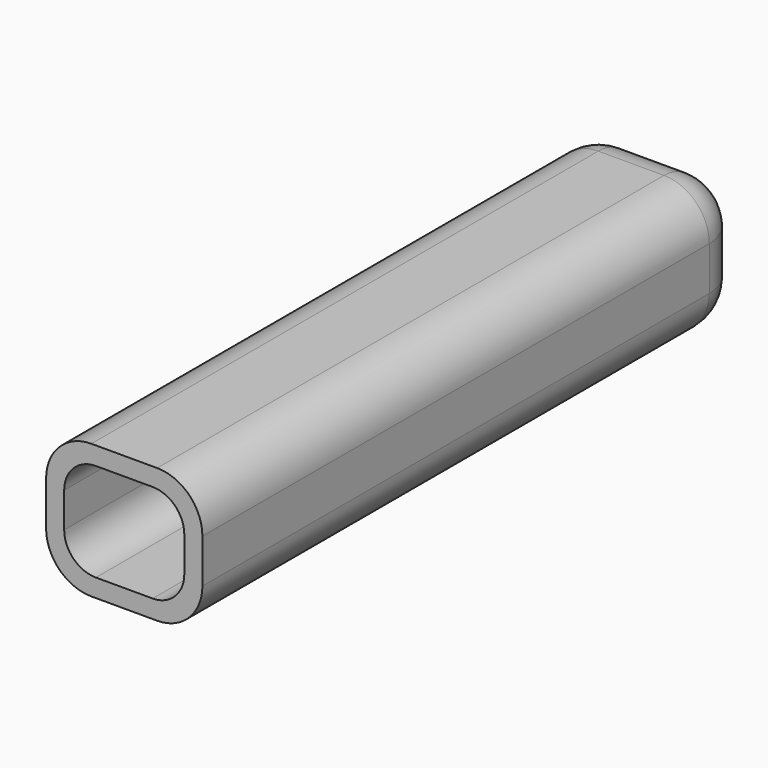
from build123d import *

# Parameters (mm, degrees)
F0_W         = 17.27
F0_H         = 14.85
F0_W_2       = 13.27
F0_H_2       = 10.85
F1_DEPTH     = 75
F2_R         = 3.5
F3_R         = 5
F4_W         = 13.27
F4_H         = 10.85
F5_DEPTH     = 5
F6_R         = 3
F7_DEPTH     = 25
F8_T1_DEPTH  = 7.27
F8_T3_DEPTH  = 4.85
F8_T6_ANGLE  = 90
F8_T8_ANGLE  = 90
F8_T10_ANGLE = 90
F8_T12_ANGLE = 90


# Not quite as in the source:
# - a fillet or chamfer that OpenCascade refuses, or shapes differently, is made with other operations: its cross-section is extruded or revolved along the edge and cut away or added


with BuildPart() as f1:
    # F0 (on Front) → F1 (new body)
    with BuildSketch(Plane.XZ):
        with Locations((6.635, 5.425)):
            Rectangle(F0_W, F0_H)
        with Locations((6.635, 5.425)):
            Rectangle(F0_W_2, F0_H_2, mode=Mode.SUBTRACT)
    extrude(amount=F1_DEPTH)

    # F2
    f2_edges = [f1.edges().sort_by_distance(p)[0] for p in [
        (0, -37.5, 10.85),
        (13.27, -37.5, 0),
        (13.27, -37.5, 10.85),
        (0, -37.5, 0),
    ]]
    fillet(f2_edges, radius=F2_R)

    # F3
    f3_edges = [f1.edges().sort_by_distance(p)[0] for p in [
        (-2, -37.5, 12.85),
        (15.27, -37.5, 12.85),
        (15.27, -37.5, -2),
        (-2, -37.5, -2),
    ]]
    fillet(f3_edges, radius=F3_R)

    # F4 (on face) → F5 (join)
    with BuildSketch(Plane.XZ):
        with Locations((6.635, 5.425)):
            Rectangle(F4_W, F4_H)
    extrude(amount=F5_DEPTH)

    # F6 (on face) → F7 (cut)
    with BuildSketch(Plane.XZ):
        with Locations((6.635, 5.425)):
            Circle(F6_R)
    extrude(amount=F7_DEPTH, mode=Mode.SUBTRACT)

    # F8: fillet of radius 5 on 8 edges, made by hand

    # F8_s2 → F8_t1 (cut)
    with BuildSketch(Plane.YZ.offset(3)):
        with BuildLine():
            ThreePointArc((0, 7.85), (-1.4644660941, 11.3855339059), (-5, 12.85))
            Line((-5, 12.85), (0, 12.85))
            Line((0, 12.85), (0, 7.85))
        make_face()
        with BuildLine():
            ThreePointArc((0, 3), (-1.4644660941, -0.5355339059), (-5, -2))
            Line((-5, -2), (0, -2))
            Line((0, -2), (0, 3))
        make_face()
    extrude(amount=F8_T1_DEPTH, mode=Mode.SUBTRACT)

    # F8_s4 → F8_t3 (cut)
    with BuildSketch(Plane.XY.offset(3)):
        with BuildLine():
            ThreePointArc((3, 0), (-0.5355339059, -1.4644660941), (-2, -5))
            Line((-2, -5), (-2, 0))
            Line((-2, 0), (3, 0))
        make_face()
        with BuildLine():
            ThreePointArc((10.27, 0), (13.8055339059, -1.4644660941), (15.27, -5))
            Line((15.27, -5), (15.27, 0))
            Line((15.27, 0), (10.27, 0))
        make_face()
    extrude(amount=F8_T3_DEPTH, mode=Mode.SUBTRACT)

    # F8_s5 → F8_t6 (revolve, cut)
    with BuildSketch(Plane.XY.offset(7.85)):
        with BuildLine():
            ThreePointArc((3, 0), (-0.5355339059, -1.4644660941), (-2, -5))
            Line((-2, -5), (-2, 0))
            Line((-2, 0), (3, 0))
        make_face()
    revolve(axis=Axis((3, 0, 7.85), (0, 1, 0)), revolution_arc=F8_T6_ANGLE, mode=Mode.SUBTRACT)

    # F8_s7 → F8_t8 (revolve, cut)
    with BuildSketch(Plane.XY.offset(3)):
        with BuildLine():
            ThreePointArc((3, 0), (-0.5355339059, -1.4644660941), (-2, -5))
            Line((-2, -5), (-2, 0))
            Line((-2, 0), (3, 0))
        make_face()
    revolve(axis=Axis((3, 0, 3), (0, -1, 0)), revolution_arc=F8_T8_ANGLE, mode=Mode.SUBTRACT)

    # F8_s9 → F8_t10 (revolve, cut)
    with BuildSketch(Plane.XY.offset(7.85)):
        with BuildLine():
            ThreePointArc((10.27, 0), (13.8055339059, -1.4644660941), (15.27, -5))
            Line((15.27, -5), (15.27, 0))
            Line((15.27, 0), (10.27, 0))
        make_face()
    revolve(axis=Axis((10.27, 0, 7.85), (0, -1, 0)), revolution_arc=F8_T10_ANGLE, mode=Mode.SUBTRACT)

    # F8_s11 → F8_t12 (revolve, cut)
    with BuildSketch(Plane.YZ.offset(10.27)):
        with BuildLine():
            ThreePointArc((0, 3), (-1.4644660941, -0.5355339059), (-5, -2))
            Line((-5, -2), (0, -2))
            Line((0, -2), (0, 3))
        make_face()
    revolve(axis=Axis((10.27, 0, 3), (0, -1, 0)), revolution_arc=F8_T12_ANGLE, mode=Mode.SUBTRACT)


solid = f1.part
